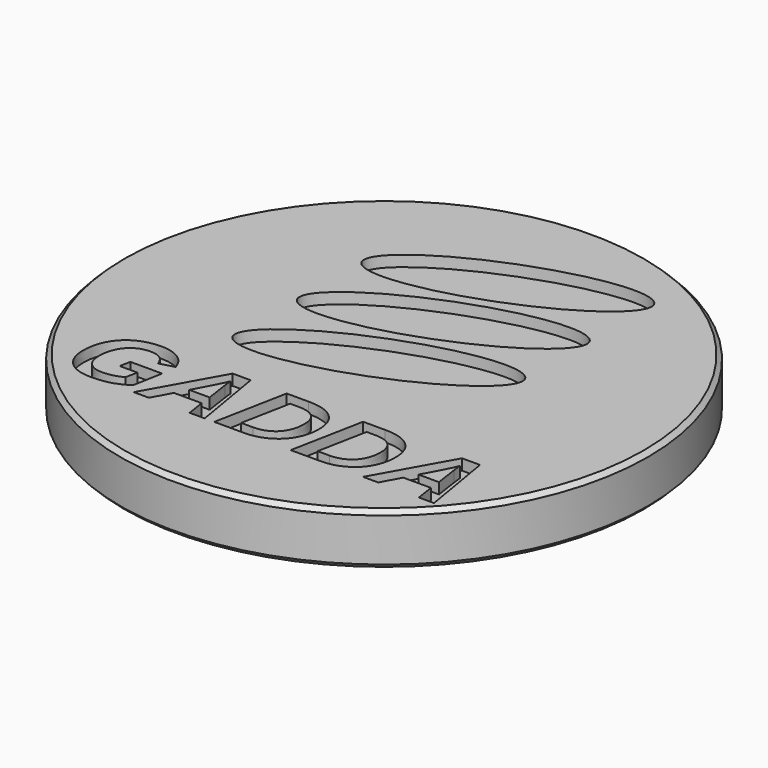
from build123d import *

# Parameters (mm, degrees)
F1_R         = 12.125
F2_DEPTH     = 2.38
F3_SIZE      = 0.2
F4_TEXT_SIZE = 4.8621370175
F5_DEPTH     = 0.5
F6_TEXT_SIZE = 5.6143067518
F7_DEPTH     = 0.5


# Not quite as in the source:
# - Text() gives the source's letters only with a copy of the font that has no kerning and outlines rounded to 1/6400 em; it was checked with that copy


with BuildPart() as f2:
    # F1 (on Top) → F2 (new body)
    with BuildSketch(Plane.XY):
        Circle(F1_R)
    extrude(amount=F2_DEPTH)

    # F3
    f3_edges = [f2.edges().sort_by_distance(p)[0] for p in [
        (-12.125, 0, 2.38),
        (-12.125, 0, 0),
    ]]
    chamfer(f3_edges, length=F3_SIZE)

    # F4 (on face) → F5 (cut)
    with BuildSketch(Plane.XY.offset(2.38)):
        with BuildLine():
            add(Edge.make_bspline(
                [(5.1412415081, 9.0576154836), (4.2182739379, 11.486222258), (-3.0321045391, 7.3411032079), (-10.2824830161, 3.1959841577), (-2.109136969, 4.9124964335), (6.0642090782, 6.6290087093), (5.1412415081, 9.0576154836)],
                knots=[0, 0, 0, 2.0943951024, 2.0943951024, 4.1887902048, 4.1887902048, 6.2831853072, 6.2831853072, 6.2831853072], degree=2, weights=[1, 0.5, 1, 0.5, 1, 0.5, 1]))
        make_face()
        with BuildLine():
            add(Edge.make_bspline(
                [(5.1412415081, 5.3538771086), (4.2182739379, 7.782483883), (-3.0321045391, 3.6373648329), (-10.2824830161, -0.5077542173), (-2.109136969, 1.2087580585), (6.0642090782, 2.9252703343), (5.1412415081, 5.3538771086)],
                knots=[0, 0, 0, 2.0943951024, 2.0943951024, 4.1887902048, 4.1887902048, 6.2831853072, 6.2831853072, 6.2831853072], degree=2, weights=[1, 0.5, 1, 0.5, 1, 0.5, 1]))
        make_face()
        with BuildLine():
            add(Edge.make_bspline(
                [(5.1412415081, 1.6501387336), (4.2182739379, 4.078745508), (-3.0321045391, -0.0663735422), (-10.2824830161, -4.2114925923), (-2.109136969, -2.4949803165), (6.0642090782, -0.7784680407), (5.1412415081, 1.6501387336)],
                knots=[0, 0, 0, 2.0943951024, 2.0943951024, 4.1887902048, 4.1887902048, 6.2831853072, 6.2831853072, 6.2831853072], degree=2, weights=[1, 0.5, 1, 0.5, 1, 0.5, 1]))
        make_face()
        with Locations((-8.8705063637, -7.889189708)):
            Text('GADDA', F4_TEXT_SIZE, font='Arimo', font_style=FontStyle.BOLDITALIC, text_align=(TextAlign.LEFT, TextAlign.BOTTOM))
    extrude(amount=-F5_DEPTH, mode=Mode.SUBTRACT)

    # F6 (on face) → F7 (cut)
    with BuildSketch(Plane(origin=(0, 0, 0), x_dir=(1, 0, 0), z_dir=(0, 0, -1))):
        with BuildLine():
            add(Edge.make_bspline(
                [(-5.2990314417, -0.7688928974), (-4.6031333298, -3.272036085), (2.9974647768, 0.1893088013), (10.5980628834, 3.6506536876), (2.3015666649, 2.6924519889), (-5.9949295537, 1.7342502902), (-5.2990314417, -0.7688928974)],
                knots=[0, 0, 0, 2.0943951024, 2.0943951024, 4.1887902048, 4.1887902048, 6.2831853072, 6.2831853072, 6.2831853072], degree=2, weights=[1, 0.5, 1, 0.5, 1, 0.5, 1]))
        make_face()
        with BuildLine():
            add(Edge.make_bspline(
                [(-5.2990314417, 3.0583438473), (-4.6031333298, 0.5552006597), (2.9974647768, 4.016545546), (10.5980628834, 7.4778904323), (2.3015666649, 6.5196887336), (-5.9949295537, 5.561487035), (-5.2990314417, 3.0583438473)],
                knots=[0, 0, 0, 2.0943951024, 2.0943951024, 4.1887902048, 4.1887902048, 6.2831853072, 6.2831853072, 6.2831853072], degree=2, weights=[1, 0.5, 1, 0.5, 1, 0.5, 1]))
        make_face()
        with BuildLine():
            add(Edge.make_bspline(
                [(-5.2990314417, 6.8855805921), (-4.6031333298, 4.3824374045), (2.9974647768, 7.8437822908), (10.5980628834, 11.3051271771), (2.3015666649, 10.3469254784), (-5.9949295537, 9.3887237797), (-5.2990314417, 6.8855805921)],
                knots=[0, 0, 0, 2.0943951024, 2.0943951024, 4.1887902048, 4.1887902048, 6.2831853072, 6.2831853072, 6.2831853072], degree=2, weights=[1, 0.5, 1, 0.5, 1, 0.5, 1]))
        make_face()
        with Locations((-9.229099378, -6.7315476481)):
            Text('GADDA', F6_TEXT_SIZE, font='Open Sans', font_style=FontStyle.BOLDITALIC, text_align=(TextAlign.LEFT, TextAlign.BOTTOM))
    extrude(amount=-F7_DEPTH, mode=Mode.SUBTRACT)


solid = f2.part
